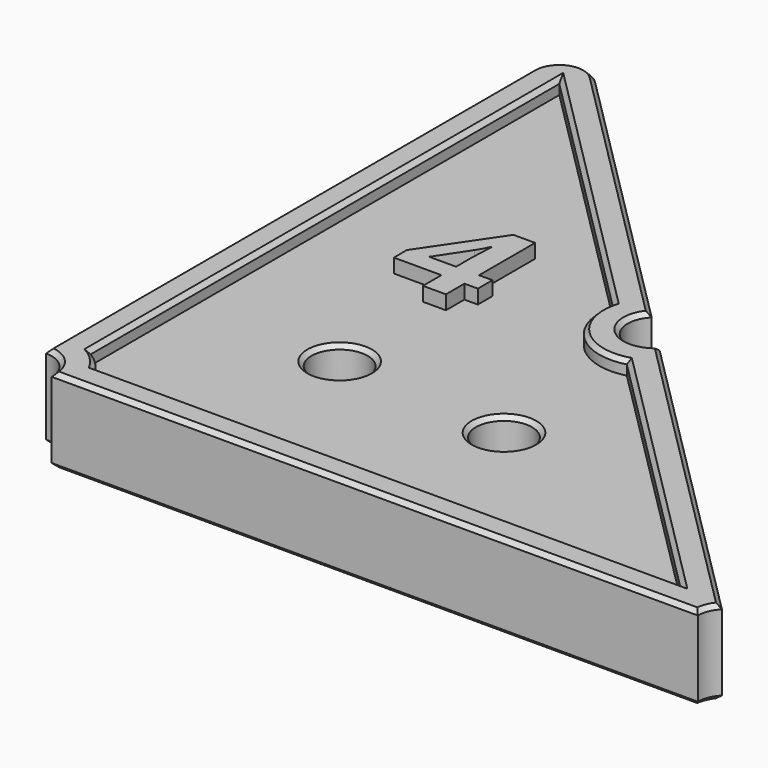
from build123d import *

# Parameters (mm, degrees)
F0_R         = 2
F0_TEXT_SIZE = 11.1111111111
F1_DEPTH     = 5
F3_DEPTH     = 1
F4_SIZE      = 0.3


# Not quite as in the source:
# - Text() gives the source's letters only with a copy of the font that has no kerning and outlines rounded to 1/6400 em; it was checked with that copy


with BuildPart() as f1:
    # F0 (on Top) → F1 (new body)
    with BuildSketch(Plane.XY):
        with BuildLine():
            ThreePointArc((-21.5857864376, 21.5857864376), (-23.7653668647, 22.0193319403), (-25, 20.1715728753))
            Line((-25, 20.1715728753), (-25, -23))
            ThreePointArc((-25, -23), (-23.5857864376, -23.5857864376), (-23, -25))
            Line((-23, -25), (23, -25))
            ThreePointArc((23, -25), (23.152240935, -24.2346331353), (23.5857864376, -23.5857864376))
            Line((23.5857864376, -23.5857864376), (1.4142135624, -1.4142135624))
            ThreePointArc((1.4142135624, -1.4142135624), (-1.4142135624, -1.4142135624), (-1.4142135624, 1.4142135624))
            Line((-1.4142135624, 1.4142135624), (-21.5857864376, 21.5857864376))
        make_face()
        with Locations((-12.5, -12.5)):
            Circle(F0_R, mode=Mode.SUBTRACT)
        with Locations((0, -13.5)):
            Circle(F0_R, mode=Mode.SUBTRACT)
        Polygon((-10.7760416667, -1.0538194444), (-10.7760416667, -2.3559027778), (-11.7309027778, -2.3559027778), (-11.7309027778, -4), (-13.3697916667, -4), (-13.3697916667, -2.3559027778), (-16.7552083333, -2.3559027778), (-16.7552083333, -1.1892361111), (-13.2760416667, 3.9322916667), (-11.7309027778, 3.9322916667), (-11.7309027778, -1.0538194444), align=None, mode=Mode.SUBTRACT)
        with Locations((-16.9444444444, -4)):
            Text('4', F0_TEXT_SIZE, font='Open Sans', font_style=FontStyle.BOLD, text_align=(TextAlign.LEFT, TextAlign.BOTTOM))
        with BuildLine():
            Line((-15.2795138889, -1.0538194444), (-13.3697916667, -1.0538194444))
            Line((-13.3697916667, -1.0538194444), (-13.3697916667, 0.2916666667))
            add(Edge.make_bspline(
                [(-13.3697916667, 0.2916666667), (-13.3697916667, 0.6284722222), (-13.3420138889, 1.2682291667)],
                knots=[0, 0, 0, 1, 1, 1], degree=2))
            add(Edge.make_bspline(
                [(-13.3420138889, 1.2682291667), (-13.3142361111, 1.9079861111), (-13.2986111111, 2.0121527778)],
                knots=[0, 0, 0, 1, 1, 1], degree=2))
            Line((-13.2986111111, 2.0121527778), (-13.3420138889, 2.0121527778))
            add(Edge.make_bspline(
                [(-13.3420138889, 2.0121527778), (-13.5434027778, 1.5659722222), (-13.8246527778, 1.1440972222)],
                knots=[0, 0, 0, 1, 1, 1], degree=2))
            Line((-13.8246527778, 1.1440972222), (-15.2795138889, -1.0538194444))
        make_face()
    extrude(amount=-F1_DEPTH)

    # F0 (on Top) + F2 (on face) → F3 (join)
    with BuildSketch(Plane.XY):
        with Locations((-16.9444444444, -4)):
            Text('4', F0_TEXT_SIZE, font='Open Sans', font_style=FontStyle.BOLD, text_align=(TextAlign.LEFT, TextAlign.BOTTOM))
    with BuildSketch(Plane.XY):
        with BuildLine():
            ThreePointArc((1.4142135624, -1.4142135624), (-1.4142135624, -1.4142135624), (-1.4142135624, 1.4142135624))
            Line((-1.4142135624, 1.4142135624), (-21.5857864376, 21.5857864376))
            ThreePointArc((-21.5857864376, 21.5857864376), (-23.7653668647, 22.0193319403), (-25, 20.1715728753))
            Line((-25, 20.1715728753), (-25, -23))
            ThreePointArc((-25, -23), (-23.5857864376, -23.5857864376), (-23, -25))
            Line((-23, -25), (23, -25))
            ThreePointArc((23, -25), (23.152240935, -24.2346331353), (23.5857864376, -23.5857864376))
            Line((23.5857864376, -23.5857864376), (1.4142135624, -1.4142135624))
        make_face()
        with BuildLine():
            Line((1.0352761804, -3.8637033052), (20.1715728753, -23))
            Line((20.1715728753, -23), (-21.5358983849, -23))
            ThreePointArc((-21.5358983849, -23), (-22.1715728753, -22.1715728753), (-23, -21.5358983849))
            Line((-23, -21.5358983849), (-23, 20.1715728753))
            Line((-23, 20.1715728753), (-3.8637033052, 1.0352761804))
            ThreePointArc((-3.8637033052, 1.0352761804), (-2.8284271247, -2.8284271247), (1.0352761804, -3.8637033052))
        make_face(mode=Mode.SUBTRACT)
    extrude(amount=F3_DEPTH)

    # F4
    f4_edges = [f1.edges().sort_by_distance(p)[0] for p in [
        (-1.414214, -1.414214, 1),
        (-11.5, 11.5, 1),
        (-23.765367, 22.019332, 1),
        (-25, -1.414214, 1),
        (-23.585786, -23.585786, 1),
        (0, -25, 1),
        (23.152241, -24.234633, 1),
        (12.5, -12.5, 1),
        (-13.431852, 10.603425, 1),
        (-2.828427, -2.828427, 1),
        (10.603425, -13.431852, 1),
        (-0.682163, -23, 1),
        (-22.171573, -22.171573, 1),
        (-23, -0.682163, 1),
        (-14.5, -12.5, 0),
        (-2, -13.5, 0),
        (-11.5, 11.5, -5),
        (-23.765367, 22.019332, -5),
        (-25, -1.414214, -5),
        (-23.585786, -23.585786, -5),
        (0, -25, -5),
        (23.152241, -24.234633, -5),
        (12.5, -12.5, -5),
        (-1.414214, -1.414214, -5),
        (-14.5, -12.5, -5),
        (-2, -13.5, -5),
    ]]
    chamfer(f4_edges, length=F4_SIZE)


solid = f1.part
